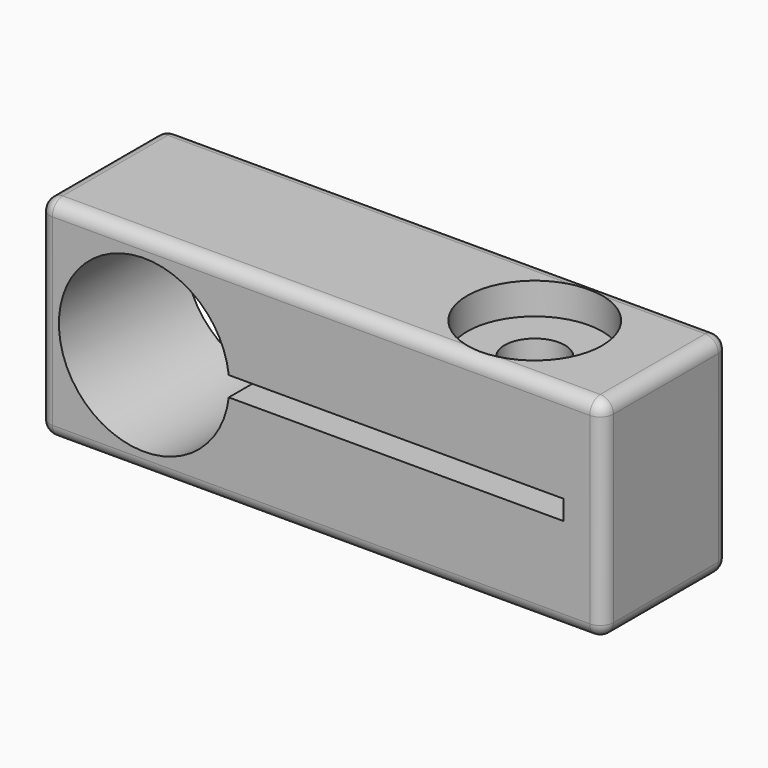
from build123d import *

# Parameters (mm, degrees)
F0_W         = 43
F0_H         = 16
F1_DEPTH     = 6
F2_R         = 2.3
F3_DEPTH     = 16
F2_R_2       = 5.15
F4_DEPTH     = 2.4
F5_R         = 2.3
F6_DEPTH     = 3
F7_T1_DEPTH  = 10
F7_T3_DEPTH  = 41
F7_T5_DEPTH  = 14
F7_S9_W      = 1
F7_S9_H      = 1
F7_T10_DEPTH = 1
F7_S15_W     = 1
F7_S15_H     = 1
F7_T16_DEPTH = 1
F7_S21_W     = 1
F7_S21_H     = 1
F7_T22_DEPTH = 1
F7_S27_W     = 1
F7_S27_H     = 1
F7_T28_DEPTH = 1
F7_S33_W     = 1
F7_S33_H     = 1
F7_T34_DEPTH = 1
F7_S39_W     = 1
F7_S39_H     = 1
F7_T40_DEPTH = 1
F7_S45_W     = 1
F7_S45_H     = 1
F7_T46_DEPTH = 1
F7_S51_W     = 1
F7_S51_H     = 1
F7_T52_DEPTH = 1


# Not quite as in the source:
# - a fillet or chamfer that OpenCascade refuses, or shapes differently, is made with other operations: its cross-section is extruded or revolved along the edge and cut away or added


with BuildPart() as f1:
    # F0 (on Front) → F1 (new body, symmetric)
    with BuildSketch(Plane.XZ):
        Rectangle(F0_W, F0_H)
        with BuildLine():
            ThreePointArc((-7.0434142149, -0.75), (-20, 0), (-7.0434142149, 0.75))
            Line((-7.0434142149, 0.75), (18.5, 0.75))
            Line((18.5, 0.75), (18.5, -0.75))
            Line((18.5, -0.75), (-7.0434142149, -0.75))
        make_face(mode=Mode.SUBTRACT)
    extrude(amount=F1_DEPTH, both=True)

    # F2 (on face) → F3 (cut, through all)
    with BuildSketch(Plane.XY.offset(8)):
        with Locations((11.5, 0)):
            Circle(F2_R)
    extrude(amount=-F3_DEPTH, mode=Mode.SUBTRACT)

    # F2 (on face) → F4 (cut)
    with BuildSketch(Plane.XY.offset(8)):
        with Locations((11.5, 0)):
            Circle(F2_R_2)
        with Locations((11.5, 0)):
            Circle(F2_R, mode=Mode.SUBTRACT)
    extrude(amount=-F4_DEPTH, mode=Mode.SUBTRACT)

    # F5 (on face) → F6 (cut)
    with BuildSketch(Plane(origin=(0, 0, -8), x_dir=(1, 0, 0), z_dir=(0, 0, -1))):
        Polygon((13.5784609691, 3.6), (9.4215390309, 3.6), (7.3430780618, 0), (9.4215390309, -3.6), (13.5784609691, -3.6), (15.6569219382, 0), align=None)
        with Locations((11.5, 0)):
            Circle(F5_R, mode=Mode.SUBTRACT)
    extrude(amount=-F6_DEPTH, mode=Mode.SUBTRACT)

    # F7: fillet of radius 1 on 12 edges, made by hand

    # F7_s2 → F7_t1 (cut)
    with BuildSketch(Plane.XZ.offset(-5)):
        with BuildLine():
            ThreePointArc((-21.5, -7), (-21.2071067812, -7.7071067812), (-20.5, -8))
            Line((-20.5, -8), (-21.5, -8))
            Line((-21.5, -8), (-21.5, -7))
        make_face()
        with BuildLine():
            ThreePointArc((21.5, -7), (21.2071067812, -7.7071067812), (20.5, -8))
            Line((20.5, -8), (21.5, -8))
            Line((21.5, -8), (21.5, -7))
        make_face()
        with BuildLine():
            ThreePointArc((-20.5, 8), (-21.2071067812, 7.7071067812), (-21.5, 7))
            Line((-21.5, 7), (-21.5, 8))
            Line((-21.5, 8), (-20.5, 8))
        make_face()
        with BuildLine():
            ThreePointArc((20.5, 8), (21.2071067812, 7.7071067812), (21.5, 7))
            Line((21.5, 7), (21.5, 8))
            Line((21.5, 8), (20.5, 8))
        make_face()
    extrude(amount=F7_T1_DEPTH, mode=Mode.SUBTRACT)

    # F7_s4 → F7_t3 (cut)
    with BuildSketch(Plane.YZ.offset(-20.5)):
        with BuildLine():
            ThreePointArc((-6, -7), (-5.7071067812, -7.7071067812), (-5, -8))
            Line((-5, -8), (-6, -8))
            Line((-6, -8), (-6, -7))
        make_face()
        with BuildLine():
            ThreePointArc((6, -7), (5.7071067812, -7.7071067812), (5, -8))
            Line((5, -8), (6, -8))
            Line((6, -8), (6, -7))
        make_face()
        with BuildLine():
            ThreePointArc((-5, 8), (-5.7071067812, 7.7071067812), (-6, 7))
            Line((-6, 7), (-6, 8))
            Line((-6, 8), (-5, 8))
        make_face()
        with BuildLine():
            ThreePointArc((5, 8), (5.7071067812, 7.7071067812), (6, 7))
            Line((6, 7), (6, 8))
            Line((6, 8), (5, 8))
        make_face()
    extrude(amount=F7_T3_DEPTH, mode=Mode.SUBTRACT)

    # F7_s6 → F7_t5 (cut)
    with BuildSketch(Plane.XY.offset(-7)):
        with BuildLine():
            ThreePointArc((20.5, 6), (21.2071067812, 5.7071067812), (21.5, 5))
            Line((21.5, 5), (21.5, 6))
            Line((21.5, 6), (20.5, 6))
        make_face()
        with BuildLine():
            ThreePointArc((21.5, -5), (21.2071067812, -5.7071067812), (20.5, -6))
            Line((20.5, -6), (21.5, -6))
            Line((21.5, -6), (21.5, -5))
        make_face()
        with BuildLine():
            ThreePointArc((-20.5, 6), (-21.2071067812, 5.7071067812), (-21.5, 5))
            Line((-21.5, 5), (-21.5, 6))
            Line((-21.5, 6), (-20.5, 6))
        make_face()
        with BuildLine():
            ThreePointArc((-21.5, -5), (-21.2071067812, -5.7071067812), (-20.5, -6))
            Line((-20.5, -6), (-21.5, -6))
            Line((-21.5, -6), (-21.5, -5))
        make_face()
    extrude(amount=F7_T5_DEPTH, mode=Mode.SUBTRACT)


with BuildPart() as f7_tool8:
    # F7_s9 → F7_t10 (new body)
    with BuildSketch(Plane.XZ.offset(-5)):
        with Locations((-21, -7.5)):
            Rectangle(F7_S9_W, F7_S9_H)
    extrude(amount=-F7_T10_DEPTH)

    # F7_s11 → F7_t12 (revolve, cut)
    with BuildSketch(Plane(origin=(-20.5, 5, -7), x_dir=(0.7071067812, 0, 0.7071067812), z_dir=(-0.7071067812, 0, 0.7071067812))):
        with BuildLine():
            ThreePointArc((0, -1), (1, 0), (0, 1))
            Line((0, 1), (0, -1))
        make_face()
    revolve(axis=Axis((-20.5, 5, -7), (0, 1, 0)), mode=Mode.SUBTRACT)


with BuildPart() as f1_1:
    add(f1.part)

    # F7_t7: cut F7_tool8
    add(f7_tool8.part, mode=Mode.SUBTRACT)


with BuildPart() as f7_tool14:
    # F7_s15 → F7_t16 (new body)
    with BuildSketch(Plane.YZ.offset(-20.5)):
        with Locations((-5.5, -7.5)):
            Rectangle(F7_S15_W, F7_S15_H)
    extrude(amount=-F7_T16_DEPTH)

    # F7_s17 → F7_t18 (revolve, cut)
    with BuildSketch(Plane(origin=(-20.5, -5, -7), x_dir=(0, 0.7071067812, 0.7071067812), z_dir=(0, -0.7071067812, 0.7071067812))):
        with BuildLine():
            ThreePointArc((0, -1), (1, 0), (0, 1))
            Line((0, 1), (0, -1))
        make_face()
    revolve(axis=Axis((-20.5, -5, -7), (-1, 0, 0)), mode=Mode.SUBTRACT)


with BuildPart() as f1_2:
    add(f1_1.part)

    # F7_t13: cut F7_tool14
    add(f7_tool14.part, mode=Mode.SUBTRACT)


with BuildPart() as f7_tool20:
    # F7_s21 → F7_t22 (new body)
    with BuildSketch(Plane.YZ.offset(20.5)):
        with Locations((-5.5, -7.5)):
            Rectangle(F7_S21_W, F7_S21_H)
    extrude(amount=F7_T22_DEPTH)

    # F7_s23 → F7_t24 (revolve, cut)
    with BuildSketch(Plane(origin=(20.5, -5, -7), x_dir=(0, 0.7071067812, 0.7071067812), z_dir=(0, 0.7071067812, -0.7071067812))):
        with BuildLine():
            ThreePointArc((0, -1), (1, 0), (0, 1))
            Line((0, 1), (0, -1))
        make_face()
    revolve(axis=Axis((20.5, -5, -7), (1, 0, 0)), mode=Mode.SUBTRACT)


with BuildPart() as f1_3:
    add(f1_2.part)

    # F7_t19: cut F7_tool20
    add(f7_tool20.part, mode=Mode.SUBTRACT)


with BuildPart() as f7_tool26:
    # F7_s27 → F7_t28 (new body)
    with BuildSketch(Plane.XZ.offset(-5)):
        with Locations((21, -7.5)):
            Rectangle(F7_S27_W, F7_S27_H)
    extrude(amount=-F7_T28_DEPTH)

    # F7_s29 → F7_t30 (revolve, cut)
    with BuildSketch(Plane(origin=(20.5, 5, -7), x_dir=(-0.7071067812, 0, 0.7071067812), z_dir=(-0.7071067812, 0, -0.7071067812))):
        with BuildLine():
            ThreePointArc((0, -1), (1, 0), (0, 1))
            Line((0, 1), (0, -1))
        make_face()
    revolve(axis=Axis((20.5, 5, -7), (0, 1, 0)), mode=Mode.SUBTRACT)


with BuildPart() as f1_4:
    add(f1_3.part)

    # F7_t25: cut F7_tool26
    add(f7_tool26.part, mode=Mode.SUBTRACT)


with BuildPart() as f7_tool32:
    # F7_s33 → F7_t34 (new body)
    with BuildSketch(Plane.XY.offset(7)):
        with Locations((21, 5.5)):
            Rectangle(F7_S33_W, F7_S33_H)
    extrude(amount=F7_T34_DEPTH)

    # F7_s35 → F7_t36 (revolve, cut)
    with BuildSketch(Plane(origin=(20.5, 5, 7), x_dir=(-0.7071067812, -0.7071067812, 0), z_dir=(-0.7071067812, 0.7071067812, 0))):
        with BuildLine():
            ThreePointArc((0, -1), (1, 0), (0, 1))
            Line((0, 1), (0, -1))
        make_face()
    revolve(axis=Axis((20.5, 5, 7), (0, 0, 1)), mode=Mode.SUBTRACT)


with BuildPart() as f1_5:
    add(f1_4.part)

    # F7_t31: cut F7_tool32
    add(f7_tool32.part, mode=Mode.SUBTRACT)


with BuildPart() as f7_tool38:
    # F7_s39 → F7_t40 (new body)
    with BuildSketch(Plane.XY.offset(7)):
        with Locations((21, -5.5)):
            Rectangle(F7_S39_W, F7_S39_H)
    extrude(amount=F7_T40_DEPTH)

    # F7_s41 → F7_t42 (revolve, cut)
    with BuildSketch(Plane(origin=(20.5, -5, 7), x_dir=(-0.7071067812, 0.7071067812, 0), z_dir=(0.7071067812, 0.7071067812, 0))):
        with BuildLine():
            ThreePointArc((0, -1), (1, 0), (0, 1))
            Line((0, 1), (0, -1))
        make_face()
    revolve(axis=Axis((20.5, -5, 7), (0, 0, 1)), mode=Mode.SUBTRACT)


with BuildPart() as f1_6:
    add(f1_5.part)

    # F7_t37: cut F7_tool38
    add(f7_tool38.part, mode=Mode.SUBTRACT)


with BuildPart() as f7_tool44:
    # F7_s45 → F7_t46 (new body)
    with BuildSketch(Plane.XY.offset(7)):
        with Locations((-21, 5.5)):
            Rectangle(F7_S45_W, F7_S45_H)
    extrude(amount=F7_T46_DEPTH)

    # F7_s47 → F7_t48 (revolve, cut)
    with BuildSketch(Plane(origin=(-20.5, 5, 7), x_dir=(0.7071067812, -0.7071067812, 0), z_dir=(-0.7071067812, -0.7071067812, 0))):
        with BuildLine():
            ThreePointArc((0, -1), (1, 0), (0, 1))
            Line((0, 1), (0, -1))
        make_face()
    revolve(axis=Axis((-20.5, 5, 7), (0, 0, 1)), mode=Mode.SUBTRACT)


with BuildPart() as f1_7:
    add(f1_6.part)

    # F7_t43: cut F7_tool44
    add(f7_tool44.part, mode=Mode.SUBTRACT)


with BuildPart() as f7_tool50:
    # F7_s51 → F7_t52 (new body)
    with BuildSketch(Plane.XY.offset(7)):
        with Locations((-21, -5.5)):
            Rectangle(F7_S51_W, F7_S51_H)
    extrude(amount=F7_T52_DEPTH)

    # F7_s53 → F7_t54 (revolve, cut)
    with BuildSketch(Plane(origin=(-20.5, -5, 7), x_dir=(0.7071067812, 0.7071067812, 0), z_dir=(0.7071067812, -0.7071067812, 0))):
        with BuildLine():
            ThreePointArc((0, -1), (1, 0), (0, 1))
            Line((0, 1), (0, -1))
        make_face()
    revolve(axis=Axis((-20.5, -5, 7), (0, 0, 1)), mode=Mode.SUBTRACT)


with BuildPart() as f1_8:
    add(f1_7.part)

    # F7_t49: cut F7_tool50
    add(f7_tool50.part, mode=Mode.SUBTRACT)


solid = f1_8.part
